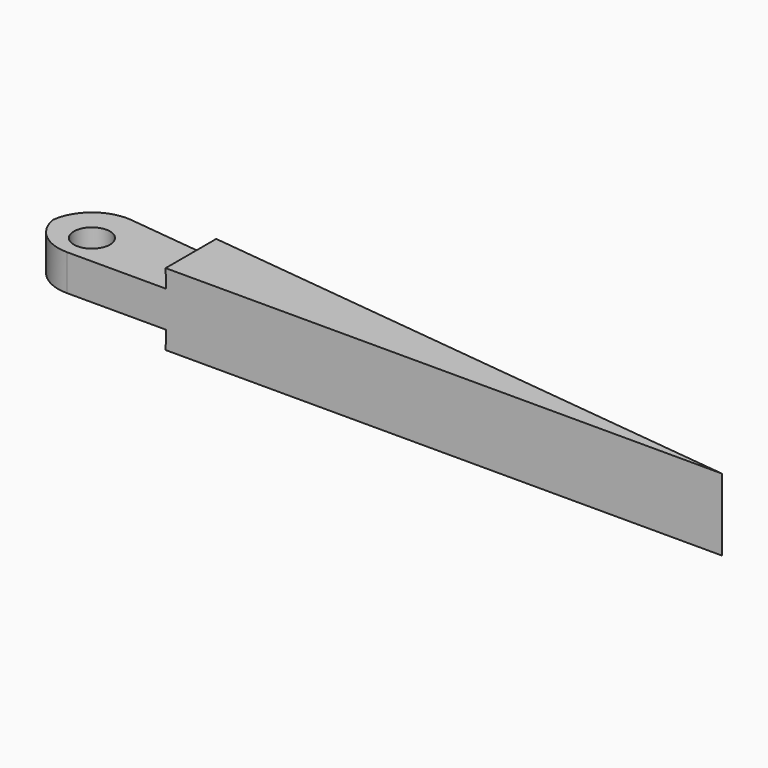
from build123d import *

# Parameters (mm, degrees)
F1_DEPTH    = 3.175
F3_DEPTH    = 25.4
F4_T1_DEPTH = 21.629832931
F4_T3_DEPTH = 25.208081251
F6_D        = 3.175


# Not quite as in the source:
# - a fillet or chamfer that OpenCascade refuses, or shapes differently, is made with other operations: its cross-section is extruded or revolved along the edge and cut away or added


with BuildPart() as f1:
    # F0 (on Top) → F1 (new body, symmetric)
    with BuildSketch(Plane.XY):
        Polygon((-31.6706262529, 7.0008751936), (-31.4483754337, 0), (29.8926271498, 0), align=None)
    extrude(amount=F1_DEPTH, both=True)

    # F2 (on Front) → F3 (cut)
    with BuildSketch(Plane.XZ):
        Polygon((-32.3509715194, 5.2941306494), (-32.3509715194, 1.5875), (-19.0253787046, 1.5875), (-19.1175676882, 5.2941306494), align=None)
        Polygon((-19.0253787046, -1.5875), (-32.3509715194, -1.5875), (-32.3509715194, -5.2941306494), (-19.1175676882, -5.2941306494), align=None)
    extrude(amount=-F3_DEPTH, mode=Mode.SUBTRACT)

    # F4: fillet of radius 3.81 on 2 edges, made by hand

    # F4_s2 → F4_t1 (cut)
    with BuildSketch(Plane.XY.offset(-10.8149164655)):
        with BuildLine():
            ThreePointArc((-27.7574088475, 0), (-30.4083993967, 1.0735151913), (-31.5654904043, 3.6891080797))
            Line((-31.5654904043, 3.6891080797), (-31.4483754337, 0))
            Line((-31.4483754337, 0), (-27.7574088475, 0))
        make_face()
    extrude(amount=F4_T1_DEPTH, mode=Mode.SUBTRACT)

    # F4_s4 → F4_t3 (cut)
    with BuildSketch(Plane.XY.offset(-12.6040406255)):
        with BuildLine():
            ThreePointArc((-27.2922295058, 6.5029708841), (-30.3048140162, 5.5189587428), (-31.5308036019, 2.5964777998))
            Line((-31.5308036019, 2.5964777998), (-31.6706262529, 7.0008751936))
            Line((-31.6706262529, 7.0008751936), (-27.2922295058, 6.5029708841))
        make_face()
    extrude(amount=F4_T3_DEPTH, mode=Mode.SUBTRACT)

    # F6 (through all)
    with Locations(Plane(origin=(0, 0, -3.175), x_dir=(1, 0, 0), z_dir=(0, 0, -1))):
        with Locations((-27.722722045, -2.71736972)):
            Hole(F6_D / 2)


solid = f1.part
